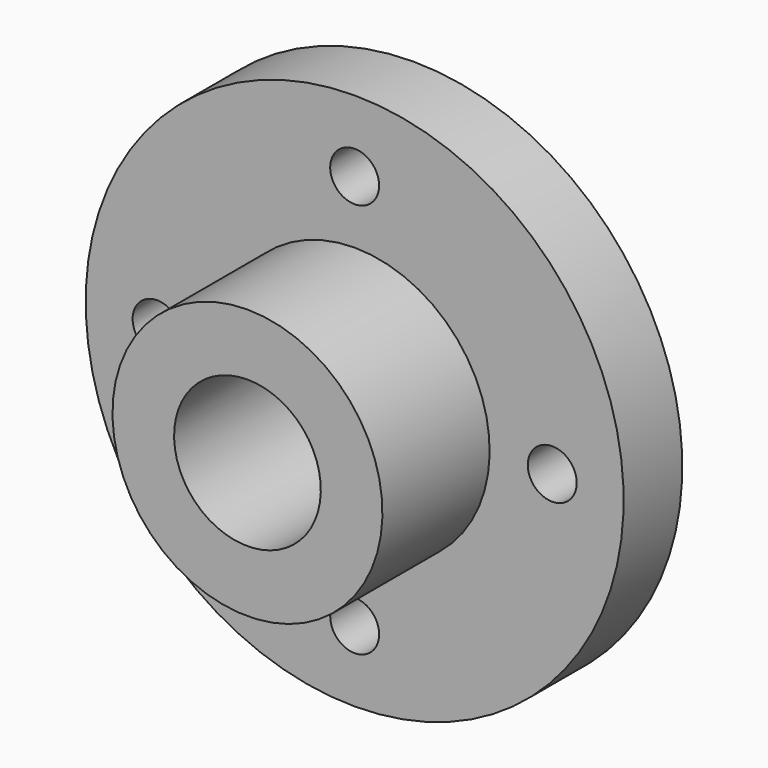
from build123d import *

# Parameters (mm, degrees)
F2_R            = 6.35
F3_DEPTH        = 53.849
F3_COPIES_COUNT = 4


# Not quite as in the source:
# - a pattern or mirror of a feature is missing from the dataset's text; its kind, count and spacing are read off the source's solid


with BuildPart() as f1:
    # F0 (on Right) → F1 (revolve)
    with BuildSketch(Plane.YZ):
        Polygon((0, 19.05), (0, 69.85), (-19.05, 69.85), (-19.05, 35.052), (-53.848, 35.052), (-53.848, 19.05), align=None)
    revolve(axis=Axis((0, -53.4342415631, 0), (0, -1, 0)))

    # F2 (on Front) → F3 (cut, through all)
    with BuildSketch(Plane.XZ):
        with Locations((0, 51.308)):
            Circle(F2_R)
    f3 = extrude(amount=F3_DEPTH, mode=Mode.SUBTRACT)

    # F3_copies: F3 ×4 about axis
    f3_copies_axis = Axis((0, 0, 0), (0, 1, 0))
    for i in range(1, F3_COPIES_COUNT):
        add(f3.rotate(f3_copies_axis, i * 360 / F3_COPIES_COUNT), mode=Mode.SUBTRACT)


solid = f1.part
